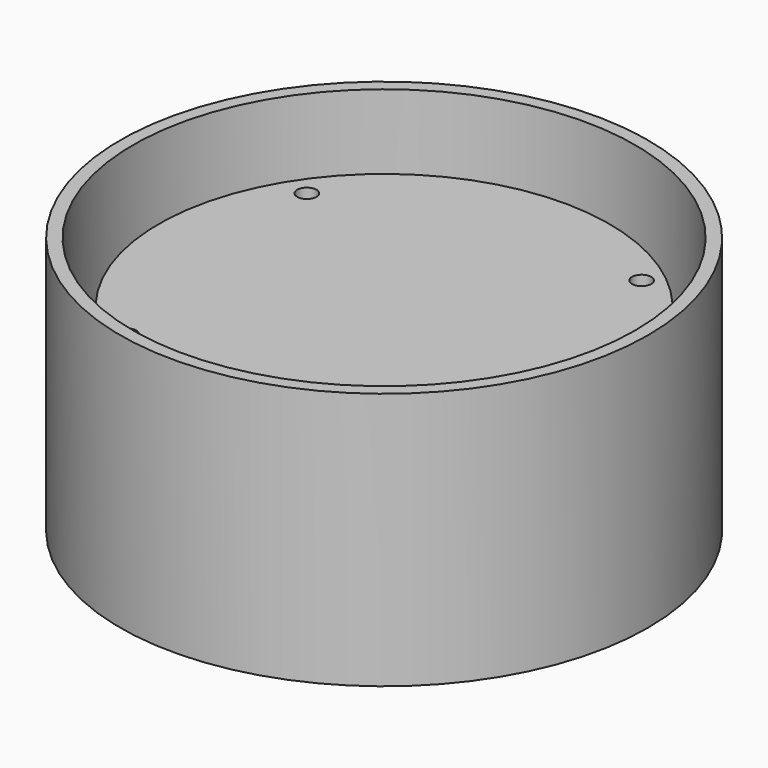
from build123d import *

# Parameters (mm, degrees)
F0_R         = 1.5
F1_DEPTH     = 1.67
F2_R         = 5
F3_DEPTH     = 9
F4_R         = 5
F6_R         = 1.5
F7_DEPTH     = 1.5
F8_R         = 1.5
F8_R_2       = 3
F9_DEPTH     = 11.83
F10_R        = 2
F11_T1_DEPTH = 5.1651459185
F13_R        = 1.5
F14_DEPTH    = 1.5
F15_R        = 1.5
F15_R_2      = 3
F16_DEPTH    = 9
F17_R        = 41
F17_R_2      = 1.5
F18_DEPTH    = 5
F19_R        = 41
F19_R_2      = 39
F20_DEPTH    = 35


# Not quite as in the source:
# - a fillet or chamfer that OpenCascade refuses, or shapes differently, is made with other operations: its cross-section is extruded or revolved along the edge and cut away or added
# - after a boolean that leaves OpenCascade's solid faulty, fix() repairs it


with BuildPart() as f1:
    # F0 (on Top) → F1 (new body)
    with BuildSketch(Plane.XY):
        with BuildLine():
            Line((-23, 12.5), (-23, -26.3818119165))
            ThreePointArc((-23, -26.3818119165), (5.4495468608, -34.5731462122), (30, -18.0277563773))
            Line((30, -18.0277563773), (30, -12.5))
            Line((30, -12.5), (23, -12.5))
            Line((23, -12.5), (23, 26.3818119165))
            ThreePointArc((23, 26.3818119165), (-5.4495468608, 34.5731462122), (-30, 18.0277563773))
            Line((-30, 18.0277563773), (-30, 12.5))
            Line((-30, 12.5), (-23, 12.5))
        make_face()
        with Locations((-20, -25)):
            Circle(F0_R, mode=Mode.SUBTRACT)
        with Locations((-18, -15.5)):
            Circle(F0_R, mode=Mode.SUBTRACT)
        with Locations((26, -17.5)):
            Circle(F0_R, mode=Mode.SUBTRACT)
        with Locations((18, -2.5)):
            Circle(F0_R, mode=Mode.SUBTRACT)
        with Locations((-18, 2.5)):
            Circle(F0_R, mode=Mode.SUBTRACT)
        with Locations((-26, 17.5)):
            Circle(F0_R, mode=Mode.SUBTRACT)
        with Locations((18, 15.5)):
            Circle(F0_R, mode=Mode.SUBTRACT)
        with Locations((20, 25)):
            Circle(F0_R, mode=Mode.SUBTRACT)
    extrude(amount=F1_DEPTH)

    # F2 (on face) → F3 (join)
    with BuildSketch(Plane(origin=(0, 0, 0), x_dir=(1, 0, 0), z_dir=(0, 0, -1))):
        with Locations((0, 29)):
            Circle(F2_R)
        with Locations((0, -29)):
            Circle(F2_R)
    extrude(amount=F3_DEPTH)

    # F4
    f4_edges = [f1.edges().sort_by_distance(p)[0] for p in [
        (-5, -29, -9),
        (-5, 29, -9),
    ]]
    fillet(f4_edges, radius=F4_R)


with BuildPart() as f7:
    # F6 (on offset) → F7 (new body)
    with BuildSketch(Plane.XY.offset(15)):
        with BuildLine():
            Line((-23, 12.5), (-23, -26.3818119165))
            ThreePointArc((-23, -26.3818119165), (5.4495468608, -34.5731462122), (30, -18.0277563773))
            Line((30, -18.0277563773), (30, -12.5))
            Line((30, -12.5), (23, -12.5))
            Line((23, -12.5), (23, 26.3818119165))
            ThreePointArc((23, 26.3818119165), (-5.4495468608, 34.5731462122), (-30, 18.0277563773))
            Line((-30, 18.0277563773), (-30, 12.5))
            Line((-30, 12.5), (-23, 12.5))
        make_face()
        with Locations((-20, -25)):
            Circle(F6_R, mode=Mode.SUBTRACT)
        with Locations((26, -17.5)):
            Circle(F6_R, mode=Mode.SUBTRACT)
        with Locations((-26, 17.5)):
            Circle(F6_R, mode=Mode.SUBTRACT)
        with Locations((20, 25)):
            Circle(F6_R, mode=Mode.SUBTRACT)
    extrude(amount=-F7_DEPTH)

    # F8 (on face) → F9 (join)
    with BuildSketch(Plane(origin=(0, 0, 13.5), x_dir=(1, 0, 0), z_dir=(0, 0, -1))):
        with BuildLine():
            Line((-23, -26.3818119165), (-23, -12.5))
            Line((-23, -12.5), (-30, -12.5))
            Line((-30, -12.5), (-30, -18.0277563773))
            ThreePointArc((-30, -18.0277563773), (-26.8271795198, -22.4789332267), (-23, -26.3818119165))
        make_face()
        with Locations((-26, -17.5)):
            Circle(F8_R, mode=Mode.SUBTRACT)
        with Locations((20, -25)):
            Circle(F8_R_2)
        with Locations((20, -25)):
            Circle(F8_R, mode=Mode.SUBTRACT)
        with Locations((-20, 25)):
            Circle(F8_R_2)
        with Locations((-20, 25)):
            Circle(F8_R, mode=Mode.SUBTRACT)
        with BuildLine():
            Line((23, 12.5), (30, 12.5))
            Line((30, 12.5), (30, 18.0277563773))
            ThreePointArc((30, 18.0277563773), (26.8271795198, 22.4789332267), (23, 26.3818119165))
            Line((23, 26.3818119165), (23, 12.5))
        make_face()
        with Locations((26, 17.5)):
            Circle(F8_R, mode=Mode.SUBTRACT)
    extrude(amount=F9_DEPTH)

    # F10
    f10_edges = [f7.edges().sort_by_distance(p)[0] for p in [
        (23, -26.381812, 7.585),
        (-23, 26.381812, 7.585),
    ]]
    fillet(f10_edges, radius=F10_R)

    # F11: fillet of radius 3 on 2 edges, made by hand

    # F11_s2 → F11_t1 (cut)
    with BuildSketch(Plane.XY.offset(13.5)):
        with BuildLine():
            ThreePointArc((-21.875, -27.321866243), (-22.7041634566, -26.2790300993), (-23, -24.9799919936))
            Line((-23, -24.9799919936), (-23, -26.3818119165))
            ThreePointArc((-23, -26.3818119165), (-22.4424225917, -26.8577301389), (-21.875, -27.321866243))
        make_face()
        with BuildLine():
            ThreePointArc((23, 24.9799919936), (22.7041634566, 26.2790300993), (21.875, 27.321866243))
            ThreePointArc((21.875, 27.321866243), (22.4424225917, 26.8577301389), (23, 26.3818119165))
            Line((23, 26.3818119165), (23, 24.9799919936))
        make_face()
    extrude(amount=F11_T1_DEPTH, mode=Mode.SUBTRACT)


with BuildPart() as f14:
    # F13 (on offset) → F14 (new body)
    with BuildSketch(Plane.XY.offset(24)):
        with BuildLine():
            ThreePointArc((-30, 18.0277563773), (6.1724408299, -34.451429204), (21.875, 27.321866243))
            ThreePointArc((21.875, 27.321866243), (-6.1724408299, 34.451429204), (-30, 18.0277563773))
        make_face()
        with Locations((-20, -25)):
            Circle(F13_R, mode=Mode.SUBTRACT)
        with Locations((26, -17.5)):
            Circle(F13_R, mode=Mode.SUBTRACT)
        with Locations((-26, 17.5)):
            Circle(F13_R, mode=Mode.SUBTRACT)
        with Locations((20, 25)):
            Circle(F13_R, mode=Mode.SUBTRACT)
    extrude(amount=F14_DEPTH)

    # F15 (on face) → F16 (join)
    with BuildSketch(Plane(origin=(0, 0, 24), x_dir=(1, 0, 0), z_dir=(0, 0, -1))):
        with BuildLine():
            Line((23, 21.5406592285), (23, 12.5))
            Line((23, 12.5), (30, 12.5))
            Line((30, 12.5), (30, 18.0277563773))
            ThreePointArc((30, 18.0277563773), (28.3600921358, 20.5110988016), (26.5151515152, 22.8461537272))
            ThreePointArc((26.5151515152, 22.8461537272), (24.3036893762, 23.4155329617), (23, 21.5406592285))
        make_face()
        with Locations((26, 17.5)):
            Circle(F15_R, mode=Mode.SUBTRACT)
        with BuildLine():
            Line((-23, -21.5406592285), (-23, -12.5))
            Line((-23, -12.5), (-30, -12.5))
            Line((-30, -12.5), (-30, -18.0277563773))
            ThreePointArc((-30, -18.0277563773), (-28.3600921358, -20.5110988016), (-26.5151515152, -22.8461537272))
            ThreePointArc((-26.5151515152, -22.8461537272), (-24.3036893762, -23.4155329617), (-23, -21.5406592285))
        make_face()
        with Locations((-26, -17.5)):
            Circle(F15_R, mode=Mode.SUBTRACT)
        with Locations((20, -25)):
            Circle(F15_R_2)
        with Locations((20, -25)):
            Circle(F15_R, mode=Mode.SUBTRACT)
        with Locations((-20, 25)):
            Circle(F15_R_2)
        with Locations((-20, 25)):
            Circle(F15_R, mode=Mode.SUBTRACT)
    extrude(amount=F16_DEPTH)


with BuildPart() as f18:
    # F17 (on face) → F18 (new body)
    with BuildSketch(Plane(origin=(0, 0, 0), x_dir=(1, 0, 0), z_dir=(0, 0, -1))):
        Circle(F17_R)
        with BuildLine():
            ThreePointArc((-36.9425229241, -12.5), (-23.0762038304, 31.4402419962), (23, 31.496031496))
            Line((23, 31.496031496), (23, 26.3818119165))
            ThreePointArc((23, 26.3818119165), (26.8271795198, 22.4789332267), (30, 18.0277563773))
            Line((30, 18.0277563773), (30, 12.5))
            Line((30, 12.5), (36.9425229241, 12.5))
            ThreePointArc((36.9425229241, 12.5), (23.0762038304, -31.4402419962), (-23, -31.496031496))
            Line((-23, -31.496031496), (-23, -26.3818119165))
            ThreePointArc((-23, -26.3818119165), (-26.8271795198, -22.4789332267), (-30, -18.0277563773))
            Line((-30, -18.0277563773), (-30, -12.5))
            Line((-30, -12.5), (-36.9425229241, -12.5))
        make_face(mode=Mode.SUBTRACT)
        with BuildLine():
            ThreePointArc((30, 18.0277563773), (26.8271795198, 22.4789332267), (23, 26.3818119165))
            Line((23, 26.3818119165), (23, 12.5))
            Line((23, 12.5), (30, 12.5))
            Line((30, 12.5), (30, 18.0277563773))
        make_face()
        with Locations((26, 17.5)):
            Circle(F17_R_2, mode=Mode.SUBTRACT)
        with BuildLine():
            Line((-23, -12.5), (-30, -12.5))
            Line((-30, -12.5), (-30, -18.0277563773))
            ThreePointArc((-30, -18.0277563773), (-26.8271795198, -22.4789332267), (-23, -26.3818119165))
            Line((-23, -26.3818119165), (-23, -12.5))
        make_face()
        with Locations((-26, -17.5)):
            Circle(F17_R_2, mode=Mode.SUBTRACT)
    extrude(amount=F18_DEPTH)

    # F19 (on face) → F20 (join)
    with BuildSketch(Plane.XY):
        Circle(F19_R)
        Circle(F19_R_2, mode=Mode.SUBTRACT)
    extrude(amount=F20_DEPTH)

    add(f18.part.fix(), mode=Mode.REPLACE)


solid = Compound([f1.part, f7.part, f14.part, f18.part])
